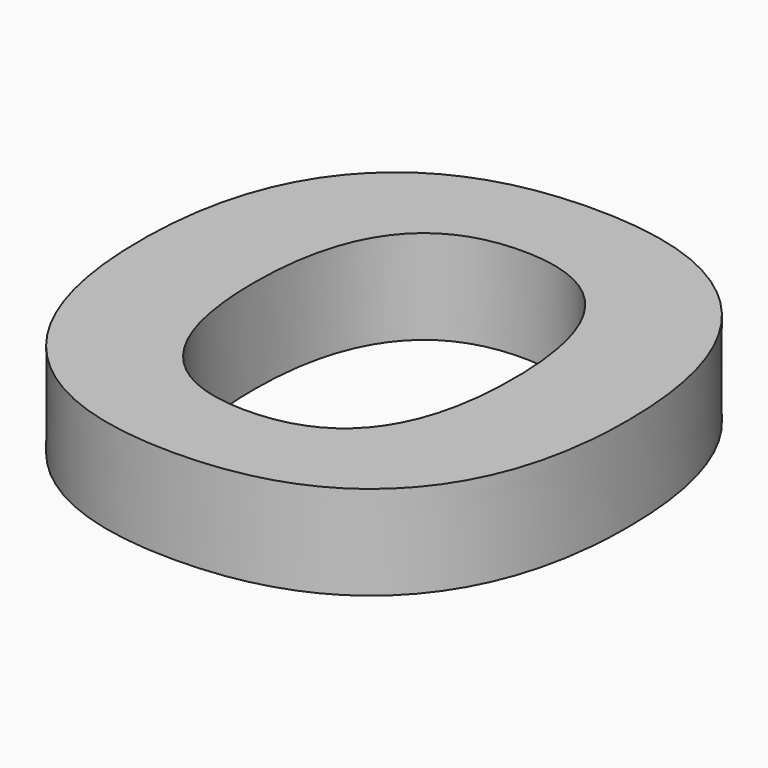
from build123d import *

# Parameters (mm, degrees)
F0_TEXT_SIZE = 76.2947990249
F1_DEPTH     = 10


# Not quite as in the source:
# - Text() gives the source's letters only with a copy of the font that has no kerning and outlines rounded to 1/6400 em; it was checked with that copy


with BuildPart() as f1:
    # F0 (on Top) → F1 (new body)
    with BuildSketch(Plane.XY):
        with Locations((0, 0)):
            Text('O', F0_TEXT_SIZE, font='Open Sans', font_style=FontStyle.BOLD, text_align=(TextAlign.LEFT, TextAlign.BOTTOM))
    extrude(amount=F1_DEPTH)


solid = f1.part
